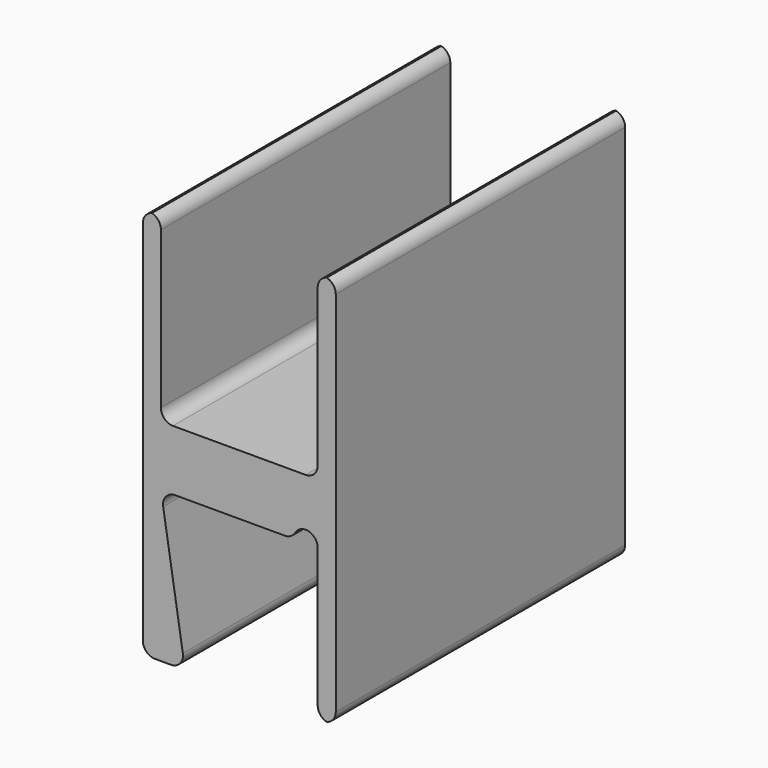
from build123d import *

# Parameters (mm, degrees)
F0_W        = 3
F0_H        = 30
F1_DEPTH    = 30
F3_DEPTH    = 60
F4_T1_DEPTH = 60
F4_T3_DEPTH = 71.7271911209
F4_T5_DEPTH = 70
F4_T7_DEPTH = 67.3205080757


# Not quite as in the source:
# - a fillet or chamfer that OpenCascade refuses, or shapes differently, is made with other operations: its cross-section is extruded or revolved along the edge and cut away or added


with BuildPart() as f1:
    # F0 (on Front) → F1 (new body, symmetric)
    with BuildSketch(Plane.XZ):
        Polygon((13, -25), (16, -25), (16, 10), (13, 10), (-13, 10), (-16, 10), (-16, -25), (-9, -25), (-13, 0), (13, 0), align=None)
        with Locations((-14.5, 25)):
            Rectangle(F0_W, F0_H)
        with Locations((14.5, 25)):
            Rectangle(F0_W, F0_H)
    extrude(amount=F1_DEPTH, both=True)

    # F2 (on face) → F3 (cut, through all)
    with BuildSketch(Plane.XZ.offset(30)):
        with BuildLine():
            Line((9, 0), (13, 0))
            ThreePointArc((13, 0), (11, 2), (9, 0))
        make_face()
    extrude(amount=-F3_DEPTH, mode=Mode.SUBTRACT)

    # F4: fillet of radius 2 on 13 edges, made by hand

    # F4_s2 → F4_t1 (join)
    with BuildSketch(Plane.XZ.offset(-30)):
        with BuildLine():
            ThreePointArc((-10.6545617758, 0), (-12.1763965245, -0.7023024244), (-12.6294430396, -2.3159810022))
            Line((-12.6294430396, -2.3159810022), (-13, 0))
            Line((-13, 0), (-10.6545617758, 0))
        make_face()
        with BuildLine():
            ThreePointArc((-13, 12), (-12.4142135624, 10.5857864376), (-11, 10))
            Line((-11, 10), (-13, 10))
            Line((-13, 10), (-13, 12))
        make_face()
        with BuildLine():
            ThreePointArc((11, 10), (12.4142135624, 10.5857864376), (13, 12))
            Line((13, 12), (13, 10))
            Line((13, 10), (11, 10))
        make_face()
    extrude(amount=F4_T1_DEPTH)

    # F4_s4 → F4_t3 (cut)
    with BuildSketch(Plane.XZ.offset(-35.8635955605)):
        with BuildLine():
            ThreePointArc((-9.3705569604, -22.6840189978), (-9.8236034755, -24.2976975756), (-11.3454382242, -25))
            Line((-11.3454382242, -25), (-9, -25))
            Line((-9, -25), (-9.3705569604, -22.6840189978))
        make_face()
    extrude(amount=F4_T3_DEPTH, mode=Mode.SUBTRACT)

    # F4_s6 → F4_t5 (cut)
    with BuildSketch(Plane.XZ.offset(-35)):
        with BuildLine():
            ThreePointArc((-14, -25), (-15.4142135624, -24.4142135624), (-16, -23))
            Line((-16, -23), (-16, -25))
            Line((-16, -25), (-14, -25))
        make_face()
        with BuildLine():
            ThreePointArc((14, -25), (15.4142135624, -24.4142135624), (16, -23))
            Line((16, -23), (16, -25))
            Line((16, -25), (14, -25))
        make_face()
        with BuildLine():
            ThreePointArc((-15, 40), (-13.5857864376, 39.4142135624), (-13, 38))
            Line((-13, 38), (-13, 40))
            Line((-13, 40), (-15, 40))
        make_face()
        with BuildLine():
            ThreePointArc((-16, 38), (-15.4142135624, 39.4142135624), (-14, 40))
            Line((-14, 40), (-16, 40))
            Line((-16, 40), (-16, 38))
        make_face()
        with BuildLine():
            ThreePointArc((16, 38), (15.4142135624, 39.4142135624), (14, 40))
            Line((14, 40), (16, 40))
            Line((16, 40), (16, 38))
        make_face()
        with BuildLine():
            ThreePointArc((13, 38), (13.5857864376, 39.4142135624), (15, 40))
            Line((15, 40), (13, 40))
            Line((13, 40), (13, 38))
        make_face()
        with BuildLine():
            ThreePointArc((15, -25), (13.5857864376, -24.4142135624), (13, -23))
            Line((13, -23), (13, -25))
            Line((13, -25), (15, -25))
        make_face()
    extrude(amount=F4_T5_DEPTH, mode=Mode.SUBTRACT)

    # F4_s8 → F4_t7 (cut)
    with BuildSketch(Plane.XZ.offset(-33.6602540378)):
        with BuildLine():
            ThreePointArc((9.2679491924, 1), (8.5358983849, 0.2679491924), (7.5358983849, 0))
            Line((7.5358983849, 0), (9, 0))
            ThreePointArc((9, 0), (9.0681483474, 0.5176380902), (9.2679491924, 1))
        make_face()
    extrude(amount=F4_T7_DEPTH, mode=Mode.SUBTRACT)


solid = f1.part
